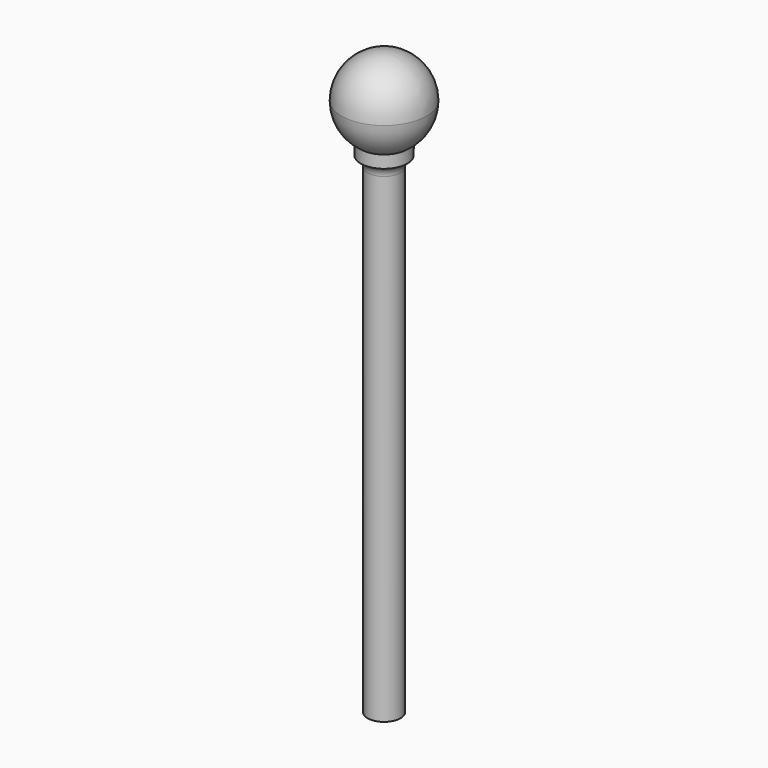
from build123d import *


# Not quite as in the source:
# - a fillet or chamfer that OpenCascade refuses, or shapes differently, is made with other operations: its cross-section is extruded or revolved along the edge and cut away or added


with BuildPart() as f1:
    # F0 (on Front) → F1 (revolve)
    with BuildSketch(Plane.XZ):
        Polygon((0, 113.175), (0, 0), (3.683, 0), (3.683, 110), (5.207, 110), (5.207, 113.175), align=None)
    revolve(axis=Axis((0, 0, 56.5875), (0, 0, -1)))

    # F2: fillet of radius 2.54 on 1 edges, made by hand

    # F2_s1 → F2_t2 (revolve)
    with BuildSketch(Plane.XZ):
        with BuildLine():
            ThreePointArc((3.683, 107.672051547), (4.0978835326, 109.063266843), (5.207, 110))
            Line((5.207, 110), (3.683, 110))
            Line((3.683, 110), (3.683, 107.672051547))
        make_face()
    revolve(axis=Axis((0, 0, 110), (0, 0, -1)))

    # F3 (on Front) → F4 (revolve)
    with BuildSketch(Plane.XZ):
        with BuildLine():
            ThreePointArc((0, 111.27), (6.7351920908, 114.0598079092), (9.525, 120.795))
            ThreePointArc((9.525, 120.795), (6.7351920908, 127.5301920908), (0, 130.32))
            Line((0, 130.32), (0, 111.27))
        make_face()
    revolve(axis=Axis((0, 0, 120.795), (0, 0, -1)))


solid = f1.part
